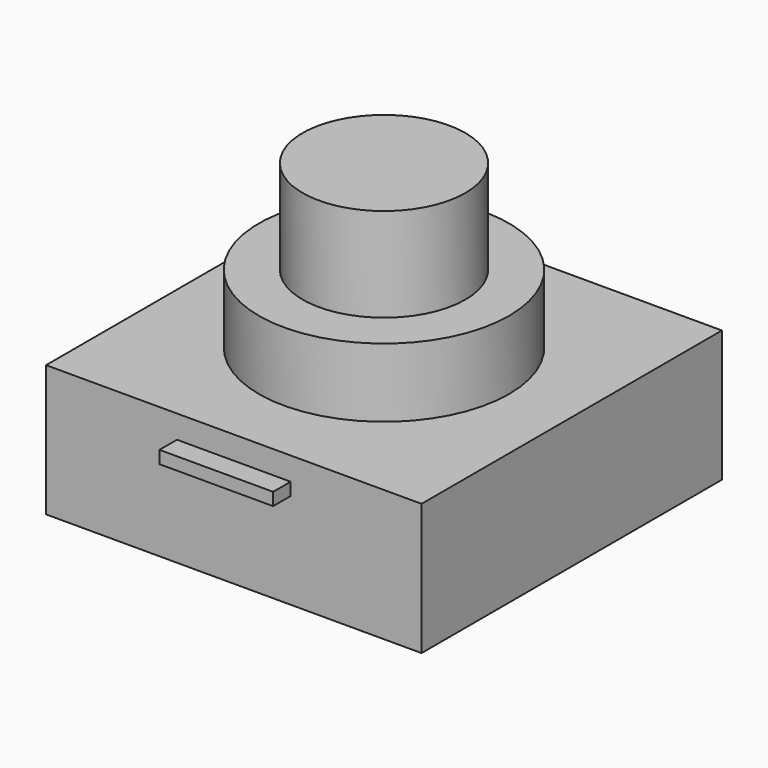
from build123d import *

# Parameters (mm, degrees)
F0_W     = 12
F0_H     = 12
F1_DEPTH = 4.2
F2_R     = 4
F3_DEPTH = 2.2
F4_R     = 2.6
F5_DEPTH = 3
F6_W     = 3.6317317281
F6_H     = 0.4035253078
F7_DEPTH = 0.7


# Not quite as in the source:
# - a pattern or mirror of a feature is missing from the dataset's text; its kind, count and spacing are read off the source's solid


with BuildPart() as f1:
    # F0 (on Top) → F1 (new body)
    with BuildSketch(Plane.XY):
        Rectangle(F0_W, F0_H)
    extrude(amount=F1_DEPTH)

    # F2 (on face) → F3 (join)
    with BuildSketch(Plane.XY.offset(4.2)):
        Circle(F2_R)
    extrude(amount=F3_DEPTH)

    # F4 (on face) → F5 (join)
    with BuildSketch(Plane.XY.offset(6.4)):
        Circle(F4_R)
    extrude(amount=F5_DEPTH)

    # F6 (on face) → F7 (join)
    with BuildSketch(Plane(origin=(0, 6, 0), x_dir=(-1, 0, 0), z_dir=(0, 1, 0))):
        with Locations((0, 3.2601370476)):
            Rectangle(F6_W, F6_H)
    f7 = extrude(amount=F7_DEPTH)

    # F7_copies: F7 across plane
    add(f7.mirror(Plane(origin=(0, 0, 0), x_dir=(0, 0, -1), z_dir=(0, -1, 0))))


solid = f1.part
